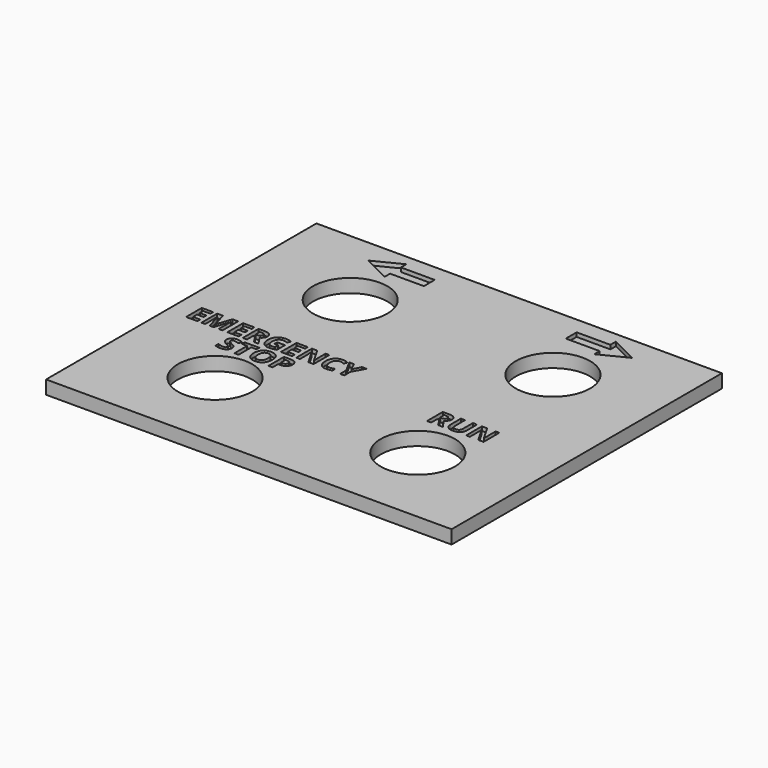
from build123d import *

# Parameters (mm, degrees)
F0_W           = 120
F0_H           = 100
F0_R           = 11
F1_DEPTH       = 4
F2_W           = 10
F2_H           = 4
F2_TEXT_SIZE   = 8.0555555556
F2_TEXT_SIZE_2 = 8.1352485064
F2_TEXT_SIZE_3 = 8.1667375585
F3_DEPTH       = 1.2


# Not quite as in the source:
# - Text() gives the source's letters only with a copy of the font that has no kerning and outlines rounded to 1/6400 em; it was checked with that copy


with BuildPart() as f1:
    # F0 (on Top) → F1 (new body)
    with BuildSketch(Plane.XY):
        Rectangle(F0_W, F0_H)
        with Locations((-30, -25)):
            Circle(F0_R, mode=Mode.SUBTRACT)
        with Locations((30, -25)):
            Circle(F0_R, mode=Mode.SUBTRACT)
        with Locations((-30, 25)):
            Circle(F0_R, mode=Mode.SUBTRACT)
        with Locations((30, 25)):
            Circle(F0_R, mode=Mode.SUBTRACT)
    extrude(amount=F1_DEPTH)

    # F2 (on face) → F3 (cut)
    with BuildSketch(Plane.XY.offset(4)):
        Polygon((-31, 45), (-31, 47), (-39, 43), (-31, 39), (-31, 41), align=None)
        with Locations((-26, 43)):
            Rectangle(F2_W, F2_H)
        with Locations((26, 43)):
            Rectangle(F2_W, F2_H)
        Polygon((39, 43), (31, 47), (31, 45), (31, 41), (31, 39), align=None)
        with Locations((-40.3658637153, -12.5784215319)):
            Text('STOP', F2_TEXT_SIZE, font='Open Sans', font_style=FontStyle.BOLD, text_align=(TextAlign.LEFT, TextAlign.BOTTOM))
        with Locations((-55, -5.3738618911)):
            Text('EMERGENCY', F2_TEXT_SIZE_2, font='Open Sans', font_style=FontStyle.BOLD, text_align=(TextAlign.LEFT, TextAlign.BOTTOM))
        with Locations((21, -11.2539129332)):
            Text('RUN', F2_TEXT_SIZE_3, font='Open Sans', font_style=FontStyle.BOLD, text_align=(TextAlign.LEFT, TextAlign.BOTTOM))
    extrude(amount=-F3_DEPTH, mode=Mode.SUBTRACT)


solid = f1.part
